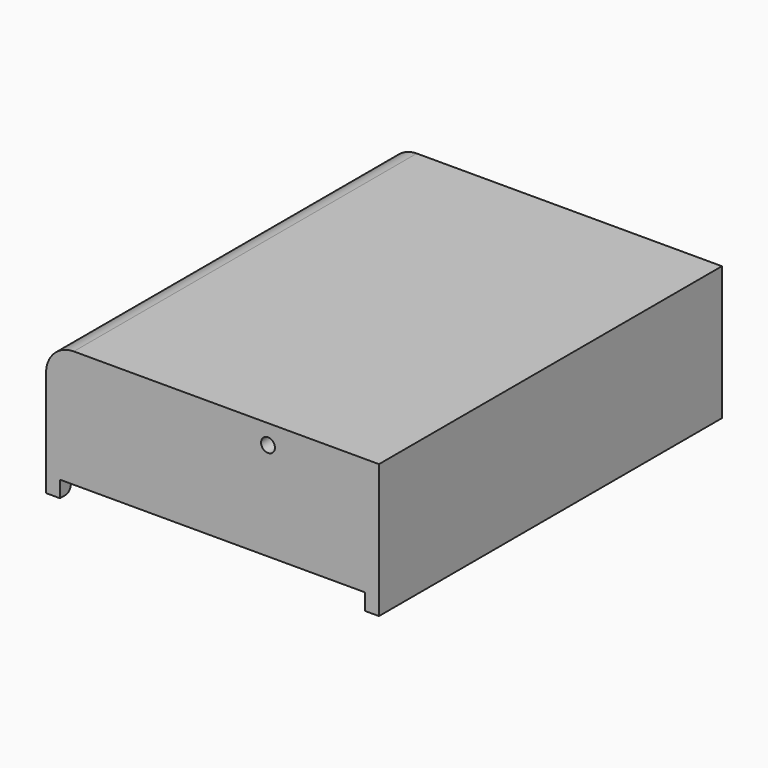
from build123d import *

# Parameters (mm, degrees)
F1_W         = 60.96
F1_H         = 78.5
F2_DEPTH     = 21.5
F0_W         = 55.88
F0_H         = 73.5
F3_DEPTH     = 19.5
F4_W         = 78.5
F4_H         = 3
F5_DEPTH     = 2.54
F6_W         = 78.5
F6_H         = 3
F7_DEPTH     = 2.54
F8_W         = 44.0962035209
F8_H         = 7.4383728206
F9_DEPTH     = 2.5
F10_W        = 5.08
F10_H        = 21.59
F11_DEPTH    = 25.4
F12_R        = 1.27
F13_R        = 1.27
F14_DEPTH    = 101.6
F15_R        = 1.27
F16_DEPTH    = 25.4
F17_T1_DEPTH = 2.54
F18_F1_R     = 5.08
F18_T2_DEPTH = 103.9


# Not quite as in the source:
# - a fillet or chamfer that OpenCascade refuses, or shapes differently, is made with other operations: its cross-section is extruded or revolved along the edge and cut away or added


with BuildPart() as f2:
    # F1 (on Top) → F2 (new body)
    with BuildSketch(Plane.XY):
        with Locations((27.94, 36.75)):
            Rectangle(F1_W, F1_H)
    extrude(amount=F2_DEPTH)

    # F0 (on Top) → F3 (cut)
    with BuildSketch(Plane.XY):
        with Locations((27.94, 36.75)):
            Rectangle(F0_W, F0_H)
    extrude(amount=F3_DEPTH, mode=Mode.SUBTRACT)

    # F4 (on face) → F5 (join, through all)
    with BuildSketch(Plane.YZ.offset(58.42)):
        with Locations((36.75, -1.5)):
            Rectangle(F4_W, F4_H)
    extrude(amount=-F5_DEPTH)

    # F6 (on face) → F7 (join, through all)
    with BuildSketch(Plane(origin=(-2.54, 0, 0), x_dir=(0, -1, 0), z_dir=(-1, 0, 0))):
        with Locations((-36.75, -1.5)):
            Rectangle(F6_W, F6_H)
    extrude(amount=-F7_DEPTH)

    # F8 (on face) → F9 (join, through all)
    with BuildSketch(Plane.XZ.offset(2.5)):
        with Locations((27.1060718223, 8.4709739313)):
            Rectangle(F8_W, F8_H)
    extrude(amount=-F9_DEPTH)

    # F10 (on face) → F11 (cut)
    with BuildSketch(Plane(origin=(-2.54, 0, 0), x_dir=(0, -1, 0), z_dir=(-1, 0, 0))):
        with Locations((-2.54, 7.795)):
            Rectangle(F10_W, F10_H)
    extrude(amount=-F11_DEPTH, mode=Mode.SUBTRACT)

    # F12
    f12_edges = [f2.edges().sort_by_distance(p)[0] for p in [
        (-1.27, 0, -3),
        (-1.27, 5.08, -3),
    ]]
    fillet(f12_edges, radius=F12_R)

    # F13 (on face) → F14 (cut)
    with BuildSketch(Plane(origin=(0, 76, 0), x_dir=(-1, 0, 0), z_dir=(0, 1, 0))):
        with Locations((-38.1, 17.955)):
            Circle(F13_R)
    extrude(amount=-F14_DEPTH, mode=Mode.SUBTRACT)

    # F15 (on face) → F16 (cut)
    with BuildSketch(Plane(origin=(-2.54, 0, 0), x_dir=(0, -1, 0), z_dir=(-1, 0, 0))):
        with Locations((-53.768, 11.605)):
            Circle(F15_R)
        with Locations((-19.732, 11.605)):
            Circle(F15_R)
    extrude(amount=-F16_DEPTH, mode=Mode.SUBTRACT)

    # F17: fillet of radius 1.27 on 2 edges, made by hand

    # F17_s2 → F17_t1 (join)
    with BuildSketch(Plane.YZ.offset(-2.54)):
        with BuildLine():
            ThreePointArc((1.2699, 18.5901), (0.3718743879, 18.2181256121), (-0.0001, 17.3201))
            Line((-0.0001, 17.3201), (-0.0255, 17.3201))
            ThreePointArc((-0.0255, 17.3201), (-0.0254, 17.95505), (-0.0254, 18.59))
            Line((-0.0254, 18.59), (0, 18.6154))
            ThreePointArc((0, 18.6154), (0.63495, 18.6154), (1.2699, 18.6155))
            Line((1.2699, 18.6155), (1.2699, 18.5901))
        make_face()
        with BuildLine():
            ThreePointArc((5.0801, 17.3201), (4.7081256121, 18.2181256121), (3.8101, 18.5901))
            Line((3.8101, 18.5901), (3.8101, 18.6155))
            ThreePointArc((3.8101, 18.6155), (4.44505, 18.6154), (5.08, 18.6154))
            Line((5.08, 18.6154), (5.1054, 18.59))
            ThreePointArc((5.1054, 18.59), (5.1054, 17.95505), (5.1055, 17.3201))
            Line((5.1055, 17.3201), (5.0801, 17.3201))
        make_face()
    extrude(amount=F17_T1_DEPTH)

    # F18: fillet of radius 5.08 on 2 edges, made by hand

    # F18_f1
    f18_f1_edges = [f2.edges().sort_by_distance(p)[0] for p in [
        (0, 36.75, 19.5),
    ]]
    fillet(f18_f1_edges, radius=F18_F1_R)

    # F18_s3 → F18_t2 (cut)
    with BuildSketch(Plane.XZ.offset(-88.7)):
        with BuildLine():
            ThreePointArc((-2.54, 16.42), (-1.0521024484, 20.0121024484), (2.54, 21.5))
            Line((2.54, 21.5), (2.54, 21.6016))
            Line((2.54, 21.6016), (-2.6416, 21.6016))
            Line((-2.6416, 21.6016), (-2.6416, 16.42))
            Line((-2.6416, 16.42), (-2.54, 16.42))
        make_face()
    extrude(amount=F18_T2_DEPTH, mode=Mode.SUBTRACT)


solid = f2.part
